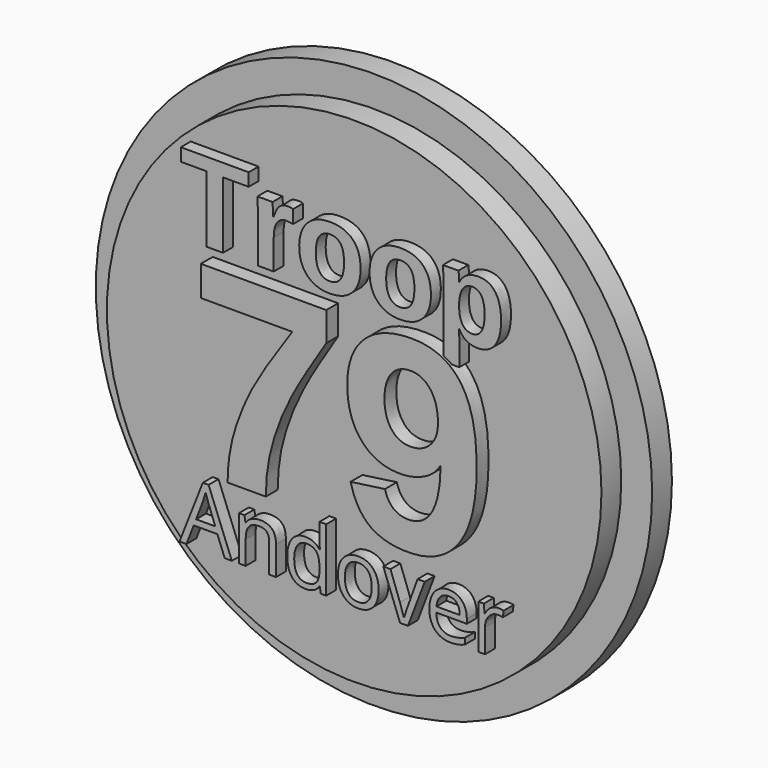
from build123d import *

# Parameters (mm, degrees)
F1_R         = 25.4
F2_DEPTH     = 2.54
F0_R         = 28.575
F3_DEPTH     = 2.54
F5_TEXT_SIZE = 11.8332953813
F7_DEPTH     = 3.81
F4_TEXT_SIZE = 27.4532409902
F8_DEPTH     = 1.524
F6_TEXT_SIZE = 8.4977443137
F9_DEPTH     = 3.81


# Not quite as in the source:
# - Text() gives the source's letters only with a copy of the font that has no kerning and outlines rounded to 1/6400 em; it was checked with that copy


with BuildPart() as f2:
    # F1 (on Front) → F2 (new body)
    with BuildSketch(Plane.XZ):
        Circle(F1_R)
    extrude(amount=F2_DEPTH)

    # F0 (on Front) → F3 (join)
    with BuildSketch(Plane.XZ):
        Circle(F0_R)
    extrude(amount=-F3_DEPTH)

    # F5 (on Front) → F7 (join)
    with BuildSketch(Plane.XZ):
        with Locations((-16.9262347763, 9.8730800673)):
            Text('Troop', F5_TEXT_SIZE, font='Arimo', font_style=FontStyle.BOLD, text_align=(TextAlign.LEFT, TextAlign.BOTTOM))
    extrude(amount=F7_DEPTH)

    # F4 (on face) → F8 (join)
    with BuildSketch(Plane.XZ.offset(2.54)):
        with Locations((-15.7105461135, -10.5748474598)):
            Text('79', F4_TEXT_SIZE, font='Arimo', font_style=FontStyle.BOLD, text_align=(TextAlign.LEFT, TextAlign.BOTTOM))
    extrude(amount=F8_DEPTH)

    # F6 (on Front) → F9 (join)
    with BuildSketch(Plane.XZ):
        with Locations((-16.9291, -17.6830568991)):
            Text('Andover', F6_TEXT_SIZE, font='Open Sans', text_align=(TextAlign.LEFT, TextAlign.BOTTOM))
    extrude(amount=F9_DEPTH)


solid = f2.part
